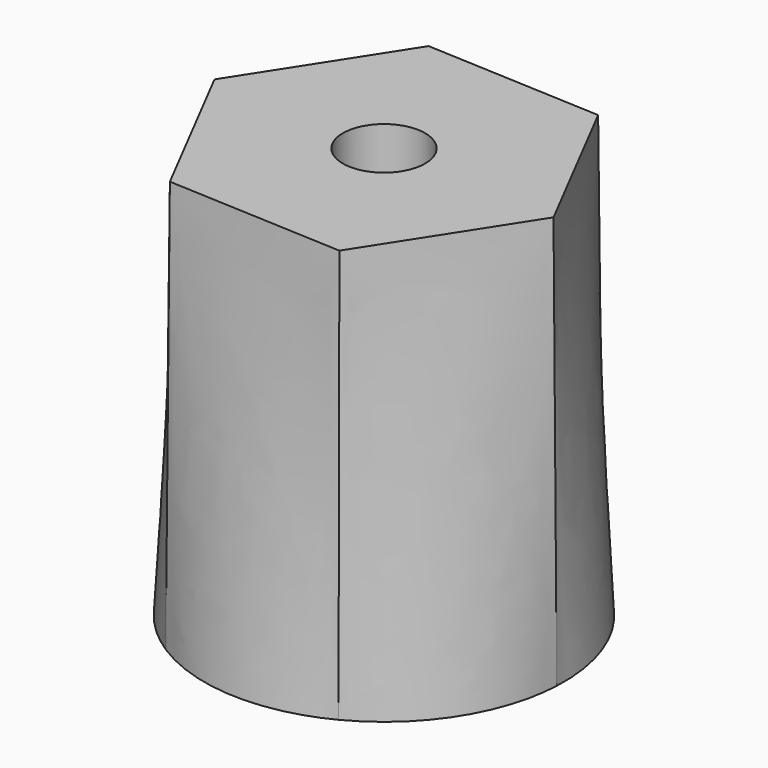
from build123d import *

# Parameters (mm, degrees)
F4_R     = 15
F5_DEPTH = 208


# Not quite as in the source:
# - the arcs of a loft's sections are written as splines that run evenly, so that the points pair up as in the source's solid


with BuildPart() as f3:
    # F2 (on offset) → F3 section 0
    with BuildSketch(Plane.XY.offset(150)):
        Polygon((29.4808263494, -57.1909035932), (64.2691885518, -3.0643072535), (34.7883622024, 54.1265963397), (-29.4808263494, 57.1909035932), (-64.2691885518, 3.0643072535), (-34.7883622024, -54.1265963397), align=None)
    # F1 (on Top) → F3 section 1
    with BuildSketch(Plane.XY):
        with BuildLine():
            add(Edge.make_bspline(
                [(30.0460333415, -58.2873687402), (33.4370549976, -56.5393613769), (36.6750958203, -54.4947096368), (42.7470280691, -49.8741177675), (45.5808257272, -47.2982489935), (50.7581543238, -41.6934743272), (53.1016053094, -38.6646549886), (57.2270197442, -32.2459957674), (59.008919485, -28.8562550072), (61.9570711279, -21.8187389434), (63.123277502, -18.1710723193), (64.8045882572, -10.7285307775), (65.319666674, -6.933770794), (65.5013587195, -3.1230562134)],
                knots=[0, 0, 0, 0, 0.1666666667, 0.1666666667, 0.3333333333, 0.3333333333, 0.5, 0.5, 0.6666666667, 0.6666666667, 0.8333333333, 0.8333333333, 1, 1, 1, 1], degree=3))
            add(Edge.make_bspline(
                [(65.5013587195, -3.1230562134), (65.683050765, 0.6876583672), (65.5313508275, 4.5142098482), (64.5657670125, 12.0829533604), (63.7518980465, 15.8250285085), (61.4866851013, 23.11111393), (60.0353761034, 26.6550116854), (56.5393613769, 33.4370549976), (54.4947096368, 36.6750958203), (49.8741177675, 42.7470280691), (47.2982489935, 45.5808257272), (41.6934743272, 50.7581543238), (38.6646549886, 53.1016053094), (35.455325378, 55.1643125268)],
                knots=[0, 0, 0, 0, 0.1666666667, 0.1666666667, 0.3333333333, 0.3333333333, 0.5, 0.5, 0.6666666667, 0.6666666667, 0.8333333333, 0.8333333333, 1, 1, 1, 1], degree=3))
            add(Edge.make_bspline(
                [(35.455325378, 55.1643125268), (32.2459957674, 57.2270197442), (28.8562550072, 59.008919485), (21.8187389434, 61.9570711279), (18.1710723193, 63.123277502), (10.7285307775, 64.8045882572), (6.933770794, 65.319666674), (-0.6876583672, 65.683050765), (-4.5142098482, 65.5313508275), (-12.0829533604, 64.5657670125), (-15.8250285085, 63.7518980465), (-23.11111393, 61.4866851013), (-26.6550116854, 60.0353761034), (-30.0460333415, 58.2873687402)],
                knots=[0, 0, 0, 0, 0.1666666667, 0.1666666667, 0.3333333333, 0.3333333333, 0.5, 0.5, 0.6666666667, 0.6666666667, 0.8333333333, 0.8333333333, 1, 1, 1, 1], degree=3))
            add(Edge.make_bspline(
                [(-30.0460333415, 58.2873687402), (-33.4370549976, 56.5393613769), (-36.6750958203, 54.4947096368), (-42.7470280691, 49.8741177675), (-45.5808257272, 47.2982489935), (-50.7581543238, 41.6934743272), (-53.1016053094, 38.6646549886), (-57.2270197442, 32.2459957674), (-59.008919485, 28.8562550072), (-61.9570711279, 21.8187389434), (-63.123277502, 18.1710723193), (-64.8045882572, 10.7285307775), (-65.319666674, 6.933770794), (-65.5013587195, 3.1230562134)],
                knots=[0, 0, 0, 0, 0.1666666667, 0.1666666667, 0.3333333333, 0.3333333333, 0.5, 0.5, 0.6666666667, 0.6666666667, 0.8333333333, 0.8333333333, 1, 1, 1, 1], degree=3))
            add(Edge.make_bspline(
                [(-65.5013587195, 3.1230562134), (-65.683050765, -0.6876583672), (-65.5313508275, -4.5142098482), (-64.5657670125, -12.0829533604), (-63.7518980465, -15.8250285085), (-61.4866851013, -23.11111393), (-60.0353761034, -26.6550116854), (-56.5393613769, -33.4370549976), (-54.4947096368, -36.6750958203), (-49.8741177675, -42.7470280691), (-47.2982489935, -45.5808257272), (-41.6934743272, -50.7581543238), (-38.6646549886, -53.1016053094), (-35.455325378, -55.1643125268)],
                knots=[0, 0, 0, 0, 0.1666666667, 0.1666666667, 0.3333333333, 0.3333333333, 0.5, 0.5, 0.6666666667, 0.6666666667, 0.8333333333, 0.8333333333, 1, 1, 1, 1], degree=3))
            add(Edge.make_bspline(
                [(-35.455325378, -55.1643125268), (-32.2459957674, -57.2270197442), (-28.8562550072, -59.008919485), (-21.8187389434, -61.9570711279), (-18.1710723193, -63.123277502), (-10.7285307775, -64.8045882572), (-6.933770794, -65.319666674), (0.6876583672, -65.683050765), (4.5142098482, -65.5313508275), (12.0829533604, -64.5657670125), (15.8250285085, -63.7518980465), (23.11111393, -61.4866851013), (26.6550116854, -60.0353761034), (30.0460333415, -58.2873687402)],
                knots=[0, 0, 0, 0, 0.1666666667, 0.1666666667, 0.3333333333, 0.3333333333, 0.5, 0.5, 0.6666666667, 0.6666666667, 0.8333333333, 0.8333333333, 1, 1, 1, 1], degree=3))
        make_face()
    loft(ruled=True)

    # F4 (on face) → F5 (cut)
    with BuildSketch(Plane(origin=(0, 0, 0), x_dir=(1, 0, 0), z_dir=(0, 0, -1))):
        Circle(F4_R)
    extrude(amount=-F5_DEPTH, mode=Mode.SUBTRACT)


solid = f3.part
